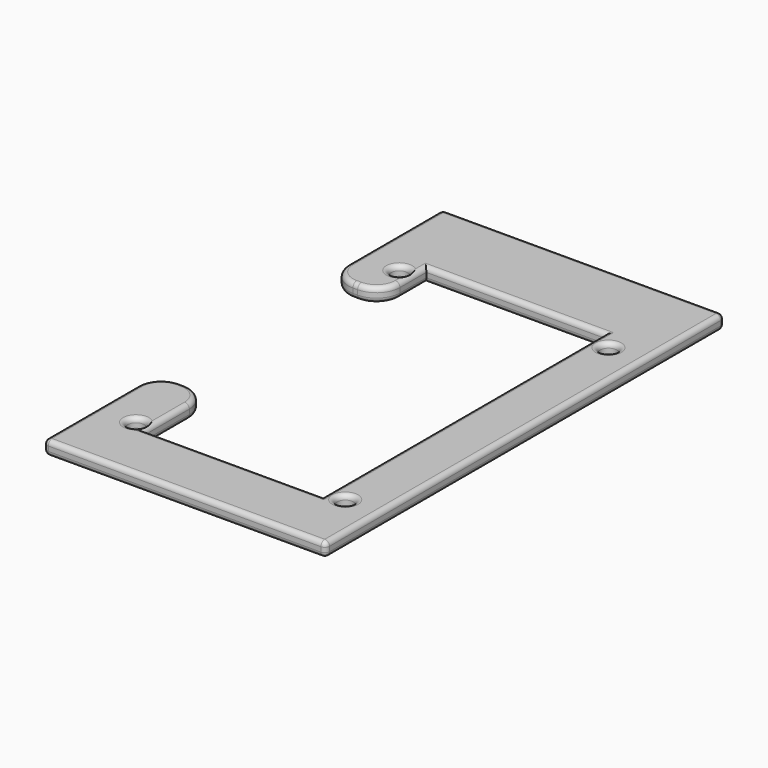
from build123d import *

# Parameters (mm, degrees)
F0_R          = 1.75
F0_W          = 38
F0_H          = 5
F1_DEPTH      = 3
F2_T1_DEPTH   = 75
F2_T3_DEPTH   = 38
F2_T5_DEPTH   = 12
F2_T7_DEPTH   = 1
F2_T9_DEPTH   = 24
F2_T11_DEPTH  = 58
F2_T13_DEPTH  = 104
F2_T15_DEPTH  = 24
F2_T17_DEPTH  = 7
F2_T19_DEPTH  = 1
F2_S23_W      = 1
F2_S23_H      = 1
F2_T24_DEPTH  = 1
F2_S29_W      = 1
F2_S29_H      = 1
F2_T30_DEPTH  = 1
F2_S35_W      = 1
F2_S35_H      = 1
F2_T36_DEPTH  = 1
F2_S41_W      = 1
F2_S41_H      = 1
F2_T42_DEPTH  = 1
F2_S47_W      = 1
F2_S47_H      = 1
F2_T48_DEPTH  = 1
F2_S53_W      = 1
F2_S53_H      = 1
F2_T54_DEPTH  = 1
F2_S59_W      = 1
F2_S59_H      = 1
F2_T60_DEPTH  = 1
F2_S65_W      = 1
F2_S65_H      = 1
F2_T66_DEPTH  = 1
F2_T70_ANGLE  = 90
F2_T72_ANGLE  = 90
F2_T74_ANGLE  = 90
F2_T76_ANGLE  = 90
F2_T86_ANGLE  = 90
F2_T88_ANGLE  = 90
F2_T90_ANGLE  = 90
F2_T92_ANGLE  = 90
F2_T105_DEPTH = 77.5
F2_T109_DEPTH = 40.5
F2_T116_DEPTH = 77.5
F2_T120_DEPTH = 40.5
F2_T127_DEPTH = 40.5
F2_T131_DEPTH = 14.5
F2_T138_DEPTH = 9.5
F2_T142_DEPTH = 40.5
F2_T149_DEPTH = 77.5
F2_T153_DEPTH = 40.5
F2_T160_DEPTH = 77.5
F2_T164_DEPTH = 40.5
F2_T171_DEPTH = 40.5
F2_T175_DEPTH = 14.5
F2_T182_DEPTH = 9.5
F2_T186_DEPTH = 40.5


# Not quite as in the source:
# - a fillet or chamfer that OpenCascade refuses, or shapes differently, is made with other operations: its cross-section is extruded or revolved along the edge and cut away or added


with BuildPart() as f1:
    # F0 (on Top) → F1 (new body)
    with BuildSketch(Plane.XY):
        with BuildLine():
            Line((17.1969585642, -33), (-20.8030414358, -33))
            Line((-20.8030414358, -33), (-20.8030414358, -29))
            Line((-20.8030414358, -29), (-20.8030414358, -21))
            ThreePointArc((-20.8030414358, -21), (-22.2675075298, -17.4644660941), (-25.8030414358, -16))
            Line((-25.8030414358, -16), (-26.8030414358, -16))
            ThreePointArc((-26.8030414358, -16), (-30.3385753417, -17.4644660941), (-31.8030414358, -21))
            Line((-31.8030414358, -21), (-31.8030414358, -46))
            Line((-31.8030414358, -46), (-26.8030414358, -46))
            Line((-26.8030414358, -46), (23.1969585642, -46))
            Line((23.1969585642, -46), (28.1969585642, -46))
            Line((28.1969585642, -46), (28.1969585642, 60))
            Line((28.1969585642, 60), (23.1969585642, 60))
            Line((23.1969585642, 60), (-26.8030414358, 60))
            Line((-26.8030414358, 60), (-31.8030414358, 60))
            Line((-31.8030414358, 60), (-31.8030414358, 35))
            ThreePointArc((-31.8030414358, 35), (-30.3385753417, 31.4644660941), (-26.8030414358, 30))
            Line((-26.8030414358, 30), (-25.8030414358, 30))
            ThreePointArc((-25.8030414358, 30), (-22.2675075298, 31.4644660941), (-20.8030414358, 35))
            Line((-20.8030414358, 35), (-20.8030414358, 42))
            Line((-20.8030414358, 42), (-20.8030414358, 47))
            Line((-20.8030414358, 47), (17.1969585642, 47))
            Line((17.1969585642, 47), (17.1969585642, 42))
            Line((17.1969585642, 42), (17.1969585642, 34))
            Line((17.1969585642, 34), (17.1969585642, -29))
            Line((17.1969585642, -29), (17.1969585642, -33))
        make_face()
        with Locations((-23.5530414358, -31.75)):
            Circle(F0_R, mode=Mode.SUBTRACT)
        with Locations((20.9469585642, -31.75)):
            Circle(F0_R, mode=Mode.SUBTRACT)
        with Locations((-23.5530414358, 38.25)):
            Circle(F0_R, mode=Mode.SUBTRACT)
        with Locations((20.9469585642, 38.25)):
            Circle(F0_R, mode=Mode.SUBTRACT)
        with Locations((-1.8030414358, 44.5)):
            Rectangle(F0_W, F0_H)
    extrude(amount=F1_DEPTH)

    # F2: fillet of radius 1 on 44 edges, made by hand

    # F2_s2 → F2_t1 (cut)
    with BuildSketch(Plane.XZ.offset(-42)):
        with BuildLine():
            ThreePointArc((17.1969585642, 2), (17.489851783, 2.7071067812), (18.1969585642, 3))
            Line((18.1969585642, 3), (17.1969585642, 3))
            Line((17.1969585642, 3), (17.1969585642, 2))
        make_face()
        with BuildLine():
            ThreePointArc((17.1969585642, 1), (17.489851783, 0.2928932188), (18.1969585642, 0))
            Line((18.1969585642, 0), (17.1969585642, 0))
            Line((17.1969585642, 0), (17.1969585642, 1))
        make_face()
    extrude(amount=F2_T1_DEPTH, mode=Mode.SUBTRACT)

    # F2_s4 → F2_t3 (cut)
    with BuildSketch(Plane.YZ.offset(-20.8030414358)):
        with BuildLine():
            ThreePointArc((-33, 2), (-33.2928932188, 2.7071067812), (-34, 3))
            Line((-34, 3), (-33, 3))
            Line((-33, 3), (-33, 2))
        make_face()
        with BuildLine():
            ThreePointArc((42, 2), (42.2928932188, 2.7071067812), (43, 3))
            Line((43, 3), (42, 3))
            Line((42, 3), (42, 2))
        make_face()
        with BuildLine():
            ThreePointArc((-33, 1), (-33.2928932188, 0.2928932188), (-34, 0))
            Line((-34, 0), (-33, 0))
            Line((-33, 0), (-33, 1))
        make_face()
        with BuildLine():
            ThreePointArc((42, 1), (42.2928932188, 0.2928932188), (43, 0))
            Line((43, 0), (42, 0))
            Line((42, 0), (42, 1))
        make_face()
    extrude(amount=F2_T3_DEPTH, mode=Mode.SUBTRACT)

    # F2_s6 → F2_t5 (cut)
    with BuildSketch(Plane.XZ.offset(21)):
        with BuildLine():
            ThreePointArc((-20.8030414358, 2), (-21.0959346546, 2.7071067812), (-21.8030414358, 3))
            Line((-21.8030414358, 3), (-20.8030414358, 3))
            Line((-20.8030414358, 3), (-20.8030414358, 2))
        make_face()
        with BuildLine():
            ThreePointArc((-20.8030414358, 1), (-21.0959346546, 0.2928932188), (-21.8030414358, 0))
            Line((-21.8030414358, 0), (-20.8030414358, 0))
            Line((-20.8030414358, 0), (-20.8030414358, 1))
        make_face()
    extrude(amount=F2_T5_DEPTH, mode=Mode.SUBTRACT)

    # F2_s8 → F2_t7 (cut)
    with BuildSketch(Plane.YZ.offset(-26.8030414358)):
        with BuildLine():
            ThreePointArc((-16, 2), (-16.2928932188, 2.7071067812), (-17, 3))
            Line((-17, 3), (-16, 3))
            Line((-16, 3), (-16, 2))
        make_face()
        with BuildLine():
            ThreePointArc((30, 2), (30.2928932188, 2.7071067812), (31, 3))
            Line((31, 3), (30, 3))
            Line((30, 3), (30, 2))
        make_face()
        with BuildLine():
            ThreePointArc((-16, 1), (-16.2928932188, 0.2928932188), (-17, 0))
            Line((-17, 0), (-16, 0))
            Line((-16, 0), (-16, 1))
        make_face()
        with BuildLine():
            ThreePointArc((30, 1), (30.2928932188, 0.2928932188), (31, 0))
            Line((31, 0), (30, 0))
            Line((30, 0), (30, 1))
        make_face()
    extrude(amount=F2_T7_DEPTH, mode=Mode.SUBTRACT)

    # F2_s10 → F2_t9 (cut)
    with BuildSketch(Plane.XZ.offset(21)):
        with BuildLine():
            ThreePointArc((-31.8030414358, 2), (-31.510148217, 2.7071067812), (-30.8030414358, 3))
            Line((-30.8030414358, 3), (-31.8030414358, 3))
            Line((-31.8030414358, 3), (-31.8030414358, 2))
        make_face()
        with BuildLine():
            ThreePointArc((-31.8030414358, 1), (-31.510148217, 0.2928932188), (-30.8030414358, 0))
            Line((-30.8030414358, 0), (-31.8030414358, 0))
            Line((-31.8030414358, 0), (-31.8030414358, 1))
        make_face()
    extrude(amount=F2_T9_DEPTH, mode=Mode.SUBTRACT)

    # F2_s12 → F2_t11 (cut)
    with BuildSketch(Plane.YZ.offset(-30.8030414358)):
        with BuildLine():
            ThreePointArc((-46, 2), (-45.7071067812, 2.7071067812), (-45, 3))
            Line((-45, 3), (-46, 3))
            Line((-46, 3), (-46, 2))
        make_face()
        with BuildLine():
            ThreePointArc((60, 2), (59.7071067812, 2.7071067812), (59, 3))
            Line((59, 3), (60, 3))
            Line((60, 3), (60, 2))
        make_face()
        with BuildLine():
            ThreePointArc((-46, 1), (-45.7071067812, 0.2928932188), (-45, 0))
            Line((-45, 0), (-46, 0))
            Line((-46, 0), (-46, 1))
        make_face()
        with BuildLine():
            ThreePointArc((60, 1), (59.7071067812, 0.2928932188), (59, 0))
            Line((59, 0), (60, 0))
            Line((60, 0), (60, 1))
        make_face()
    extrude(amount=F2_T11_DEPTH, mode=Mode.SUBTRACT)

    # F2_s14 → F2_t13 (cut)
    with BuildSketch(Plane.XZ.offset(-59)):
        with BuildLine():
            ThreePointArc((28.1969585642, 2), (27.9040653454, 2.7071067812), (27.1969585642, 3))
            Line((27.1969585642, 3), (28.1969585642, 3))
            Line((28.1969585642, 3), (28.1969585642, 2))
        make_face()
        with BuildLine():
            ThreePointArc((28.1969585642, 1), (27.9040653454, 0.2928932188), (27.1969585642, 0))
            Line((27.1969585642, 0), (28.1969585642, 0))
            Line((28.1969585642, 0), (28.1969585642, 1))
        make_face()
    extrude(amount=F2_T13_DEPTH, mode=Mode.SUBTRACT)

    # F2_s16 → F2_t15 (cut)
    with BuildSketch(Plane.XZ.offset(-59)):
        with BuildLine():
            ThreePointArc((-31.8030414358, 2), (-31.510148217, 2.7071067812), (-30.8030414358, 3))
            Line((-30.8030414358, 3), (-31.8030414358, 3))
            Line((-31.8030414358, 3), (-31.8030414358, 2))
        make_face()
        with BuildLine():
            ThreePointArc((-31.8030414358, 1), (-31.510148217, 0.2928932188), (-30.8030414358, 0))
            Line((-30.8030414358, 0), (-31.8030414358, 0))
            Line((-31.8030414358, 0), (-31.8030414358, 1))
        make_face()
    extrude(amount=F2_T15_DEPTH, mode=Mode.SUBTRACT)

    # F2_s18 → F2_t17 (cut)
    with BuildSketch(Plane.XZ.offset(-42)):
        with BuildLine():
            ThreePointArc((-20.8030414358, 2), (-21.0959346546, 2.7071067812), (-21.8030414358, 3))
            Line((-21.8030414358, 3), (-20.8030414358, 3))
            Line((-20.8030414358, 3), (-20.8030414358, 2))
        make_face()
        with BuildLine():
            ThreePointArc((-20.8030414358, 1), (-21.0959346546, 0.2928932188), (-21.8030414358, 0))
            Line((-21.8030414358, 0), (-20.8030414358, 0))
            Line((-20.8030414358, 0), (-20.8030414358, 1))
        make_face()
    extrude(amount=F2_T17_DEPTH, mode=Mode.SUBTRACT)

    # F2_s20 → F2_t19 (cut)
    with BuildSketch(Plane.XY.offset(1)):
        with BuildLine():
            ThreePointArc((28.1969585642, 59), (27.9040653454, 59.7071067812), (27.1969585642, 60))
            Line((27.1969585642, 60), (28.1969585642, 60))
            Line((28.1969585642, 60), (28.1969585642, 59))
        make_face()
        with BuildLine():
            ThreePointArc((-30.8030414358, 60), (-31.510148217, 59.7071067812), (-31.8030414358, 59))
            Line((-31.8030414358, 59), (-31.8030414358, 60))
            Line((-31.8030414358, 60), (-30.8030414358, 60))
        make_face()
        with BuildLine():
            ThreePointArc((-31.8030414358, -45), (-31.510148217, -45.7071067812), (-30.8030414358, -46))
            Line((-30.8030414358, -46), (-31.8030414358, -46))
            Line((-31.8030414358, -46), (-31.8030414358, -45))
        make_face()
        with BuildLine():
            ThreePointArc((27.1969585642, -46), (27.9040653454, -45.7071067812), (28.1969585642, -45))
            Line((28.1969585642, -45), (28.1969585642, -46))
            Line((28.1969585642, -46), (27.1969585642, -46))
        make_face()
    extrude(amount=F2_T19_DEPTH, mode=Mode.SUBTRACT)


with BuildPart() as f2_tool22:
    # F2_s23 → F2_t24 (new body)
    with BuildSketch(Plane.XY.offset(2)):
        with Locations((-31.3030414358, -45.5)):
            Rectangle(F2_S23_W, F2_S23_H)
    extrude(amount=F2_T24_DEPTH)

    # F2_s25 → F2_t26 (revolve, cut)
    with BuildSketch(Plane(origin=(-30.8030414358, -45, 2), x_dir=(0.7071067812, 0.7071067812, 0), z_dir=(0.7071067812, -0.7071067812, 0))):
        with BuildLine():
            ThreePointArc((0, -1), (1, 0), (0, 1))
            Line((0, 1), (0, -1))
        make_face()
    revolve(axis=Axis((-30.8030414358, -45, 2), (0, 0, 1)), mode=Mode.SUBTRACT)


with BuildPart() as f1_1:
    add(f1.part)

    # F2_t21: cut F2_tool22
    add(f2_tool22.part, mode=Mode.SUBTRACT)


with BuildPart() as f2_tool28:
    # F2_s29 → F2_t30 (new body)
    with BuildSketch(Plane.YZ.offset(27.1969585642)):
        with Locations((-45.5, 2.5)):
            Rectangle(F2_S29_W, F2_S29_H)
    extrude(amount=F2_T30_DEPTH)

    # F2_s31 → F2_t32 (revolve, cut)
    with BuildSketch(Plane(origin=(27.1969585642, -45, 2), x_dir=(0, 0.7071067812, -0.7071067812), z_dir=(0, -0.7071067812, -0.7071067812))):
        with BuildLine():
            ThreePointArc((0, -1), (1, 0), (0, 1))
            Line((0, 1), (0, -1))
        make_face()
    revolve(axis=Axis((27.1969585642, -45, 2), (1, 0, 0)), mode=Mode.SUBTRACT)


with BuildPart() as f1_2:
    add(f1_1.part)

    # F2_t27: cut F2_tool28
    add(f2_tool28.part, mode=Mode.SUBTRACT)


with BuildPart() as f2_tool34:
    # F2_s35 → F2_t36 (new body)
    with BuildSketch(Plane.YZ.offset(27.1969585642)):
        with Locations((59.5, 2.5)):
            Rectangle(F2_S35_W, F2_S35_H)
    extrude(amount=F2_T36_DEPTH)

    # F2_s37 → F2_t38 (revolve, cut)
    with BuildSketch(Plane(origin=(27.1969585642, 59, 2), x_dir=(0, -0.7071067812, -0.7071067812), z_dir=(0, -0.7071067812, 0.7071067812))):
        with BuildLine():
            ThreePointArc((0, -1), (1, 0), (0, 1))
            Line((0, 1), (0, -1))
        make_face()
    revolve(axis=Axis((27.1969585642, 59, 2), (1, 0, 0)), mode=Mode.SUBTRACT)


with BuildPart() as f1_3:
    add(f1_2.part)

    # F2_t33: cut F2_tool34
    add(f2_tool34.part, mode=Mode.SUBTRACT)


with BuildPart() as f2_tool40:
    # F2_s41 → F2_t42 (new body)
    with BuildSketch(Plane.XZ.offset(-59)):
        with Locations((-31.3030414358, 2.5)):
            Rectangle(F2_S41_W, F2_S41_H)
    extrude(amount=-F2_T42_DEPTH)

    # F2_s43 → F2_t44 (revolve, cut)
    with BuildSketch(Plane(origin=(-30.8030414358, 59, 2), x_dir=(0.7071067812, 0, -0.7071067812), z_dir=(0.7071067812, 0, 0.7071067812))):
        with BuildLine():
            ThreePointArc((0, -1), (1, 0), (0, 1))
            Line((0, 1), (0, -1))
        make_face()
    revolve(axis=Axis((-30.8030414358, 59, 2), (0, 1, 0)), mode=Mode.SUBTRACT)


with BuildPart() as f1_4:
    add(f1_3.part)

    # F2_t39: cut F2_tool40
    add(f2_tool40.part, mode=Mode.SUBTRACT)


with BuildPart() as f2_tool46:
    # F2_s47 → F2_t48 (new body)
    with BuildSketch(Plane.XY.offset(1)):
        with Locations((-31.3030414358, -45.5)):
            Rectangle(F2_S47_W, F2_S47_H)
    extrude(amount=-F2_T48_DEPTH)

    # F2_s49 → F2_t50 (revolve, cut)
    with BuildSketch(Plane(origin=(-30.8030414358, -45, 1), x_dir=(0.7071067812, 0.7071067812, 0), z_dir=(-0.7071067812, 0.7071067812, 0))):
        with BuildLine():
            ThreePointArc((0, -1), (1, 0), (0, 1))
            Line((0, 1), (0, -1))
        make_face()
    revolve(axis=Axis((-30.8030414358, -45, 1), (0, 0, -1)), mode=Mode.SUBTRACT)


with BuildPart() as f1_5:
    add(f1_4.part)

    # F2_t45: cut F2_tool46
    add(f2_tool46.part, mode=Mode.SUBTRACT)


with BuildPart() as f2_tool52:
    # F2_s53 → F2_t54 (new body)
    with BuildSketch(Plane.YZ.offset(27.1969585642)):
        with Locations((-45.5, 0.5)):
            Rectangle(F2_S53_W, F2_S53_H)
    extrude(amount=F2_T54_DEPTH)

    # F2_s55 → F2_t56 (revolve, cut)
    with BuildSketch(Plane(origin=(27.1969585642, -45, 1), x_dir=(0, 0.7071067812, 0.7071067812), z_dir=(0, 0.7071067812, -0.7071067812))):
        with BuildLine():
            ThreePointArc((0, -1), (1, 0), (0, 1))
            Line((0, 1), (0, -1))
        make_face()
    revolve(axis=Axis((27.1969585642, -45, 1), (1, 0, 0)), mode=Mode.SUBTRACT)


with BuildPart() as f1_6:
    add(f1_5.part)

    # F2_t51: cut F2_tool52
    add(f2_tool52.part, mode=Mode.SUBTRACT)


with BuildPart() as f2_tool58:
    # F2_s59 → F2_t60 (new body)
    with BuildSketch(Plane.YZ.offset(27.1969585642)):
        with Locations((59.5, 0.5)):
            Rectangle(F2_S59_W, F2_S59_H)
    extrude(amount=F2_T60_DEPTH)

    # F2_s61 → F2_t62 (revolve, cut)
    with BuildSketch(Plane(origin=(27.1969585642, 59, 1), x_dir=(0, -0.7071067812, 0.7071067812), z_dir=(0, 0.7071067812, 0.7071067812))):
        with BuildLine():
            ThreePointArc((0, -1), (1, 0), (0, 1))
            Line((0, 1), (0, -1))
        make_face()
    revolve(axis=Axis((27.1969585642, 59, 1), (1, 0, 0)), mode=Mode.SUBTRACT)


with BuildPart() as f1_7:
    add(f1_6.part)

    # F2_t57: cut F2_tool58
    add(f2_tool58.part, mode=Mode.SUBTRACT)


with BuildPart() as f2_tool64:
    # F2_s65 → F2_t66 (new body)
    with BuildSketch(Plane.XZ.offset(-59)):
        with Locations((-31.3030414358, 0.5)):
            Rectangle(F2_S65_W, F2_S65_H)
    extrude(amount=-F2_T66_DEPTH)

    # F2_s67 → F2_t68 (revolve, cut)
    with BuildSketch(Plane(origin=(-30.8030414358, 59, 1), x_dir=(0.7071067812, 0, 0.7071067812), z_dir=(-0.7071067812, 0, 0.7071067812))):
        with BuildLine():
            ThreePointArc((0, -1), (1, 0), (0, 1))
            Line((0, 1), (0, -1))
        make_face()
    revolve(axis=Axis((-30.8030414358, 59, 1), (0, 1, 0)), mode=Mode.SUBTRACT)


with BuildPart() as f1_8:
    add(f1_7.part)

    # F2_t63: cut F2_tool64
    add(f2_tool64.part, mode=Mode.SUBTRACT)

    # F2_s69 → F2_t70 (revolve, cut)
    with BuildSketch(Plane.XZ.offset(21)):
        with BuildLine():
            ThreePointArc((-20.8030414358, 2), (-21.0959346546, 2.7071067812), (-21.8030414358, 3))
            Line((-21.8030414358, 3), (-20.8030414358, 3))
            Line((-20.8030414358, 3), (-20.8030414358, 2))
        make_face()
    revolve(axis=Axis((-25.8030414358, -21, 3), (0, 0, 1)), revolution_arc=F2_T70_ANGLE, mode=Mode.SUBTRACT)

    # F2_s71 → F2_t72 (revolve, cut)
    with BuildSketch(Plane.YZ.offset(-26.8030414358)):
        with BuildLine():
            ThreePointArc((-16, 2), (-16.2928932188, 2.7071067812), (-17, 3))
            Line((-17, 3), (-16, 3))
            Line((-16, 3), (-16, 2))
        make_face()
    revolve(axis=Axis((-26.8030414358, -21, 3), (0, 0, 1)), revolution_arc=F2_T72_ANGLE, mode=Mode.SUBTRACT)

    # F2_s73 → F2_t74 (revolve, cut)
    with BuildSketch(Plane.XZ.offset(-35)):
        with BuildLine():
            ThreePointArc((-31.8030414358, 2), (-31.510148217, 2.7071067812), (-30.8030414358, 3))
            Line((-30.8030414358, 3), (-31.8030414358, 3))
            Line((-31.8030414358, 3), (-31.8030414358, 2))
        make_face()
    revolve(axis=Axis((-26.8030414358, 35, 3), (0, 0, 1)), revolution_arc=F2_T74_ANGLE, mode=Mode.SUBTRACT)

    # F2_s75 → F2_t76 (revolve, cut)
    with BuildSketch(Plane.YZ.offset(-25.8030414358)):
        with BuildLine():
            ThreePointArc((30, 2), (30.2928932188, 2.7071067812), (31, 3))
            Line((31, 3), (30, 3))
            Line((30, 3), (30, 2))
        make_face()
    revolve(axis=Axis((-25.8030414358, 35, 3), (0, 0, 1)), revolution_arc=F2_T76_ANGLE, mode=Mode.SUBTRACT)

    # F2_s77 → F2_t78 (revolve, cut)
    with BuildSketch(Plane.XZ.offset(31.75)):
        with BuildLine():
            ThreePointArc((-21.8030414358, 2), (-21.510148217, 2.7071067812), (-20.8030414358, 3))
            Line((-20.8030414358, 3), (-21.8030414358, 3))
            Line((-21.8030414358, 3), (-21.8030414358, 2))
        make_face()
    revolve(axis=Axis((-23.5530414358, -31.75, 3), (0, 0, 1)), mode=Mode.SUBTRACT)

    # F2_s79 → F2_t80 (revolve, cut)
    with BuildSketch(Plane.XZ.offset(31.75)):
        with BuildLine():
            ThreePointArc((22.6969585642, 2), (22.989851783, 2.7071067812), (23.6969585642, 3))
            Line((23.6969585642, 3), (22.6969585642, 3))
            Line((22.6969585642, 3), (22.6969585642, 2))
        make_face()
    revolve(axis=Axis((20.9469585642, -31.75, 3), (0, 0, 1)), mode=Mode.SUBTRACT)

    # F2_s81 → F2_t82 (revolve, cut)
    with BuildSketch(Plane.XZ.offset(-38.25)):
        with BuildLine():
            ThreePointArc((-21.8030414358, 2), (-21.510148217, 2.7071067812), (-20.8030414358, 3))
            Line((-20.8030414358, 3), (-21.8030414358, 3))
            Line((-21.8030414358, 3), (-21.8030414358, 2))
        make_face()
    revolve(axis=Axis((-23.5530414358, 38.25, 3), (0, 0, 1)), mode=Mode.SUBTRACT)

    # F2_s83 → F2_t84 (revolve, cut)
    with BuildSketch(Plane.XZ.offset(-38.25)):
        with BuildLine():
            ThreePointArc((22.6969585642, 2), (22.989851783, 2.7071067812), (23.6969585642, 3))
            Line((23.6969585642, 3), (22.6969585642, 3))
            Line((22.6969585642, 3), (22.6969585642, 2))
        make_face()
    revolve(axis=Axis((20.9469585642, 38.25, 3), (0, 0, 1)), mode=Mode.SUBTRACT)

    # F2_s85 → F2_t86 (revolve, cut)
    with BuildSketch(Plane.XZ.offset(21)):
        with BuildLine():
            ThreePointArc((-20.8030414358, 1), (-21.0959346546, 0.2928932188), (-21.8030414358, 0))
            Line((-21.8030414358, 0), (-20.8030414358, 0))
            Line((-20.8030414358, 0), (-20.8030414358, 1))
        make_face()
    revolve(axis=Axis((-25.8030414358, -21, 0), (0, 0, 1)), revolution_arc=F2_T86_ANGLE, mode=Mode.SUBTRACT)

    # F2_s87 → F2_t88 (revolve, cut)
    with BuildSketch(Plane.YZ.offset(-26.8030414358)):
        with BuildLine():
            ThreePointArc((-16, 1), (-16.2928932188, 0.2928932188), (-17, 0))
            Line((-17, 0), (-16, 0))
            Line((-16, 0), (-16, 1))
        make_face()
    revolve(axis=Axis((-26.8030414358, -21, 0), (0, 0, 1)), revolution_arc=F2_T88_ANGLE, mode=Mode.SUBTRACT)

    # F2_s89 → F2_t90 (revolve, cut)
    with BuildSketch(Plane.XZ.offset(-35)):
        with BuildLine():
            ThreePointArc((-31.8030414358, 1), (-31.510148217, 0.2928932188), (-30.8030414358, 0))
            Line((-30.8030414358, 0), (-31.8030414358, 0))
            Line((-31.8030414358, 0), (-31.8030414358, 1))
        make_face()
    revolve(axis=Axis((-26.8030414358, 35, 0), (0, 0, 1)), revolution_arc=F2_T90_ANGLE, mode=Mode.SUBTRACT)

    # F2_s91 → F2_t92 (revolve, cut)
    with BuildSketch(Plane.YZ.offset(-25.8030414358)):
        with BuildLine():
            ThreePointArc((30, 1), (30.2928932188, 0.2928932188), (31, 0))
            Line((31, 0), (30, 0))
            Line((30, 0), (30, 1))
        make_face()
    revolve(axis=Axis((-25.8030414358, 35, 0), (0, 0, 1)), revolution_arc=F2_T92_ANGLE, mode=Mode.SUBTRACT)

    # F2_s93 → F2_t94 (revolve, cut)
    with BuildSketch(Plane.XZ.offset(31.75)):
        with BuildLine():
            ThreePointArc((-21.8030414358, 1), (-21.510148217, 0.2928932188), (-20.8030414358, 0))
            Line((-20.8030414358, 0), (-21.8030414358, 0))
            Line((-21.8030414358, 0), (-21.8030414358, 1))
        make_face()
    revolve(axis=Axis((-23.5530414358, -31.75, 0), (0, 0, 1)), mode=Mode.SUBTRACT)

    # F2_s95 → F2_t96 (revolve, cut)
    with BuildSketch(Plane.XZ.offset(31.75)):
        with BuildLine():
            ThreePointArc((22.6969585642, 1), (22.989851783, 0.2928932188), (23.6969585642, 0))
            Line((23.6969585642, 0), (22.6969585642, 0))
            Line((22.6969585642, 0), (22.6969585642, 1))
        make_face()
    revolve(axis=Axis((20.9469585642, -31.75, 0), (0, 0, 1)), mode=Mode.SUBTRACT)

    # F2_s97 → F2_t98 (revolve, cut)
    with BuildSketch(Plane.XZ.offset(-38.25)):
        with BuildLine():
            ThreePointArc((-21.8030414358, 1), (-21.510148217, 0.2928932188), (-20.8030414358, 0))
            Line((-20.8030414358, 0), (-21.8030414358, 0))
            Line((-21.8030414358, 0), (-21.8030414358, 1))
        make_face()
    revolve(axis=Axis((-23.5530414358, 38.25, 0), (0, 0, 1)), mode=Mode.SUBTRACT)

    # F2_s99 → F2_t100 (revolve, cut)
    with BuildSketch(Plane.XZ.offset(-38.25)):
        with BuildLine():
            ThreePointArc((22.6969585642, 1), (22.989851783, 0.2928932188), (23.6969585642, 0))
            Line((23.6969585642, 0), (22.6969585642, 0))
            Line((22.6969585642, 0), (22.6969585642, 1))
        make_face()
    revolve(axis=Axis((20.9469585642, 38.25, 0), (0, 0, 1)), mode=Mode.SUBTRACT)


with BuildPart() as f2_tool103:
    # F2_s104 → F2_t105 (new body)
    with BuildSketch(Plane.XZ.offset(-44.5)):
        with BuildLine():
            ThreePointArc((17.1969585642, 2), (17.489851783, 2.7071067812), (18.1969585642, 3))
            Line((18.1969585642, 3), (17.1969585642, 3))
            Line((17.1969585642, 3), (17.1969585642, 2))
        make_face()
    extrude(amount=F2_T105_DEPTH)

    split(bisect_by=Plane.XZ.offset(-42), keep=Keep.BOTTOM)


with BuildPart() as f2_tool107:
    # F2_s108 → F2_t109 (new body)
    with BuildSketch(Plane.YZ.offset(-20.8030414358)):
        with BuildLine():
            ThreePointArc((42, 2), (42.2928932188, 2.7071067812), (43, 3))
            Line((43, 3), (42, 3))
            Line((42, 3), (42, 2))
        make_face()
    extrude(amount=F2_T109_DEPTH)

    split(bisect_by=Plane.YZ.offset(17.1969585642), keep=Keep.TOP)


with BuildPart() as f2_tool103_1:
    add(f2_tool103.part)

    # F2_t111: intersect F2_tool107
    add(f2_tool107.part, mode=Mode.INTERSECT)


with BuildPart() as f1_9:
    add(f1_8.part)

    # F2_t101: cut F2_tool103
    add(f2_tool103_1.part, mode=Mode.SUBTRACT)


with BuildPart() as f2_tool114:
    # F2_s115 → F2_t116 (new body)
    with BuildSketch(Plane.XZ.offset(-42)):
        with BuildLine():
            ThreePointArc((17.1969585642, 2), (17.489851783, 2.7071067812), (18.1969585642, 3))
            Line((18.1969585642, 3), (17.1969585642, 3))
            Line((17.1969585642, 3), (17.1969585642, 2))
        make_face()
    extrude(amount=F2_T116_DEPTH)

    split(bisect_by=Plane.XZ.offset(33), keep=Keep.TOP)


with BuildPart() as f2_tool118:
    # F2_s119 → F2_t120 (new body)
    with BuildSketch(Plane.YZ.offset(19.6969585642)):
        with BuildLine():
            ThreePointArc((-33, 2), (-33.2928932188, 2.7071067812), (-34, 3))
            Line((-34, 3), (-33, 3))
            Line((-33, 3), (-33, 2))
        make_face()
    extrude(amount=-F2_T120_DEPTH)

    split(bisect_by=Plane.YZ.offset(17.1969585642), keep=Keep.TOP)


with BuildPart() as f2_tool114_1:
    add(f2_tool114.part)

    # F2_t122: intersect F2_tool118
    add(f2_tool118.part, mode=Mode.INTERSECT)


with BuildPart() as f1_10:
    add(f1_9.part)

    # F2_t112: cut F2_tool114
    add(f2_tool114_1.part, mode=Mode.SUBTRACT)


with BuildPart() as f2_tool125:
    # F2_s126 → F2_t127 (new body)
    with BuildSketch(Plane.YZ.offset(17.1969585642)):
        with BuildLine():
            ThreePointArc((-33, 2), (-33.2928932188, 2.7071067812), (-34, 3))
            Line((-34, 3), (-33, 3))
            Line((-33, 3), (-33, 2))
        make_face()
    extrude(amount=-F2_T127_DEPTH)

    split(bisect_by=Plane.YZ.offset(-20.8030414358), keep=Keep.BOTTOM)


with BuildPart() as f2_tool129:
    # F2_s130 → F2_t131 (new body)
    with BuildSketch(Plane.XZ.offset(35.5)):
        with BuildLine():
            ThreePointArc((-20.8030414358, 2), (-21.0959346546, 2.7071067812), (-21.8030414358, 3))
            Line((-21.8030414358, 3), (-20.8030414358, 3))
            Line((-20.8030414358, 3), (-20.8030414358, 2))
        make_face()
    extrude(amount=-F2_T131_DEPTH)

    split(bisect_by=Plane.XZ.offset(33), keep=Keep.TOP)


with BuildPart() as f2_tool125_1:
    add(f2_tool125.part)

    # F2_t133: intersect F2_tool129
    add(f2_tool129.part, mode=Mode.INTERSECT)


with BuildPart() as f1_11:
    add(f1_10.part)

    # F2_t123: cut F2_tool125
    add(f2_tool125_1.part, mode=Mode.SUBTRACT)


with BuildPart() as f2_tool136:
    # F2_s137 → F2_t138 (new body)
    with BuildSketch(Plane.XZ.offset(-35)):
        with BuildLine():
            ThreePointArc((-20.8030414358, 2), (-21.0959346546, 2.7071067812), (-21.8030414358, 3))
            Line((-21.8030414358, 3), (-20.8030414358, 3))
            Line((-20.8030414358, 3), (-20.8030414358, 2))
        make_face()
    extrude(amount=-F2_T138_DEPTH)

    split(bisect_by=Plane.XZ.offset(-42), keep=Keep.BOTTOM)


with BuildPart() as f2_tool140:
    # F2_s141 → F2_t142 (new body)
    with BuildSketch(Plane.YZ.offset(-23.3030414358)):
        with BuildLine():
            ThreePointArc((42, 2), (42.2928932188, 2.7071067812), (43, 3))
            Line((43, 3), (42, 3))
            Line((42, 3), (42, 2))
        make_face()
    extrude(amount=F2_T142_DEPTH)

    split(bisect_by=Plane.YZ.offset(-20.8030414358), keep=Keep.BOTTOM)


with BuildPart() as f2_tool136_1:
    add(f2_tool136.part)

    # F2_t144: intersect F2_tool140
    add(f2_tool140.part, mode=Mode.INTERSECT)


with BuildPart() as f1_12:
    add(f1_11.part)

    # F2_t134: cut F2_tool136
    add(f2_tool136_1.part, mode=Mode.SUBTRACT)


with BuildPart() as f2_tool147:
    # F2_s148 → F2_t149 (new body)
    with BuildSketch(Plane.XZ.offset(-44.5)):
        with BuildLine():
            ThreePointArc((17.1969585642, 1), (17.489851783, 0.2928932188), (18.1969585642, 0))
            Line((18.1969585642, 0), (17.1969585642, 0))
            Line((17.1969585642, 0), (17.1969585642, 1))
        make_face()
    extrude(amount=F2_T149_DEPTH)

    split(bisect_by=Plane.XZ.offset(-42), keep=Keep.BOTTOM)


with BuildPart() as f2_tool151:
    # F2_s152 → F2_t153 (new body)
    with BuildSketch(Plane.YZ.offset(-20.8030414358)):
        with BuildLine():
            ThreePointArc((42, 1), (42.2928932188, 0.2928932188), (43, 0))
            Line((43, 0), (42, 0))
            Line((42, 0), (42, 1))
        make_face()
    extrude(amount=F2_T153_DEPTH)

    split(bisect_by=Plane.YZ.offset(17.1969585642), keep=Keep.TOP)


with BuildPart() as f2_tool147_1:
    add(f2_tool147.part)

    # F2_t155: intersect F2_tool151
    add(f2_tool151.part, mode=Mode.INTERSECT)


with BuildPart() as f1_13:
    add(f1_12.part)

    # F2_t145: cut F2_tool147
    add(f2_tool147_1.part, mode=Mode.SUBTRACT)


with BuildPart() as f2_tool158:
    # F2_s159 → F2_t160 (new body)
    with BuildSketch(Plane.XZ.offset(-42)):
        with BuildLine():
            ThreePointArc((17.1969585642, 1), (17.489851783, 0.2928932188), (18.1969585642, 0))
            Line((18.1969585642, 0), (17.1969585642, 0))
            Line((17.1969585642, 0), (17.1969585642, 1))
        make_face()
    extrude(amount=F2_T160_DEPTH)

    split(bisect_by=Plane.XZ.offset(33), keep=Keep.TOP)


with BuildPart() as f2_tool162:
    # F2_s163 → F2_t164 (new body)
    with BuildSketch(Plane.YZ.offset(19.6969585642)):
        with BuildLine():
            ThreePointArc((-33, 1), (-33.2928932188, 0.2928932188), (-34, 0))
            Line((-34, 0), (-33, 0))
            Line((-33, 0), (-33, 1))
        make_face()
    extrude(amount=-F2_T164_DEPTH)

    split(bisect_by=Plane.YZ.offset(17.1969585642), keep=Keep.TOP)


with BuildPart() as f2_tool158_1:
    add(f2_tool158.part)

    # F2_t166: intersect F2_tool162
    add(f2_tool162.part, mode=Mode.INTERSECT)


with BuildPart() as f1_14:
    add(f1_13.part)

    # F2_t156: cut F2_tool158
    add(f2_tool158_1.part, mode=Mode.SUBTRACT)


with BuildPart() as f2_tool169:
    # F2_s170 → F2_t171 (new body)
    with BuildSketch(Plane.YZ.offset(17.1969585642)):
        with BuildLine():
            ThreePointArc((-33, 1), (-33.2928932188, 0.2928932188), (-34, 0))
            Line((-34, 0), (-33, 0))
            Line((-33, 0), (-33, 1))
        make_face()
    extrude(amount=-F2_T171_DEPTH)

    split(bisect_by=Plane.YZ.offset(-20.8030414358), keep=Keep.BOTTOM)


with BuildPart() as f2_tool173:
    # F2_s174 → F2_t175 (new body)
    with BuildSketch(Plane.XZ.offset(35.5)):
        with BuildLine():
            ThreePointArc((-20.8030414358, 1), (-21.0959346546, 0.2928932188), (-21.8030414358, 0))
            Line((-21.8030414358, 0), (-20.8030414358, 0))
            Line((-20.8030414358, 0), (-20.8030414358, 1))
        make_face()
    extrude(amount=-F2_T175_DEPTH)

    split(bisect_by=Plane.XZ.offset(33), keep=Keep.TOP)


with BuildPart() as f2_tool169_1:
    add(f2_tool169.part)

    # F2_t177: intersect F2_tool173
    add(f2_tool173.part, mode=Mode.INTERSECT)


with BuildPart() as f1_15:
    add(f1_14.part)

    # F2_t167: cut F2_tool169
    add(f2_tool169_1.part, mode=Mode.SUBTRACT)


with BuildPart() as f2_tool180:
    # F2_s181 → F2_t182 (new body)
    with BuildSketch(Plane.XZ.offset(-35)):
        with BuildLine():
            ThreePointArc((-20.8030414358, 1), (-21.0959346546, 0.2928932188), (-21.8030414358, 0))
            Line((-21.8030414358, 0), (-20.8030414358, 0))
            Line((-20.8030414358, 0), (-20.8030414358, 1))
        make_face()
    extrude(amount=-F2_T182_DEPTH)

    split(bisect_by=Plane.XZ.offset(-42), keep=Keep.BOTTOM)


with BuildPart() as f2_tool184:
    # F2_s185 → F2_t186 (new body)
    with BuildSketch(Plane.YZ.offset(-23.3030414358)):
        with BuildLine():
            ThreePointArc((42, 1), (42.2928932188, 0.2928932188), (43, 0))
            Line((43, 0), (42, 0))
            Line((42, 0), (42, 1))
        make_face()
    extrude(amount=F2_T186_DEPTH)

    split(bisect_by=Plane.YZ.offset(-20.8030414358), keep=Keep.BOTTOM)


with BuildPart() as f2_tool180_1:
    add(f2_tool180.part)

    # F2_t188: intersect F2_tool184
    add(f2_tool184.part, mode=Mode.INTERSECT)


with BuildPart() as f1_16:
    add(f1_15.part)

    # F2_t178: cut F2_tool180
    add(f2_tool180_1.part, mode=Mode.SUBTRACT)


solid = f1_16.part
